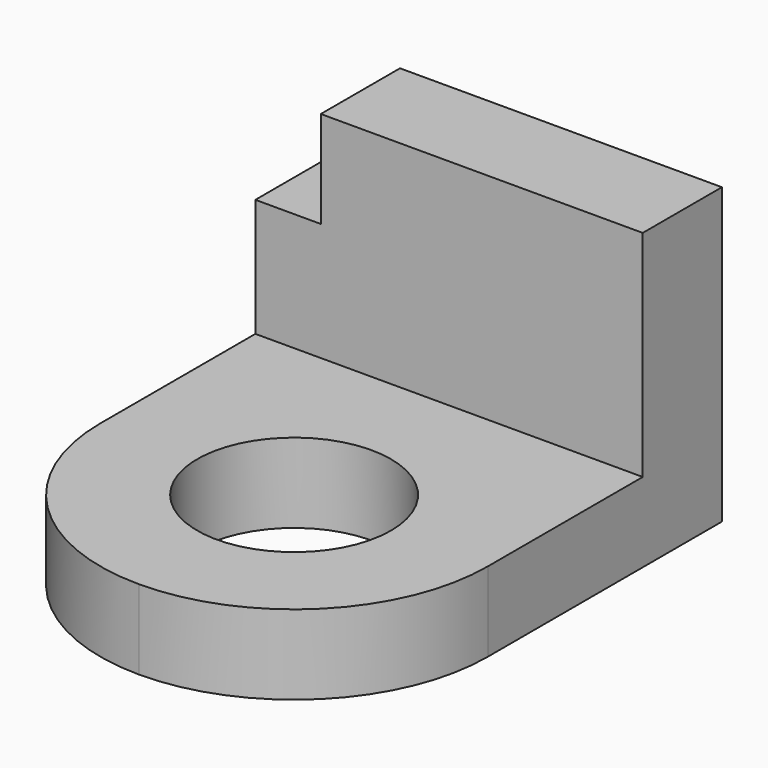
from build123d import *

# Parameters (mm, degrees)
F0_W     = 12.9794
F0_H     = 25.908
F1_DEPTH = 25.4
F2_W     = 42.2184414506
F2_H     = 12.9794
F3_DEPTH = 12.7
F4_W     = 50.8
F4_H     = 10.4306445336
F5_DEPTH = 50.8
F6_R     = 12.7
F7_DEPTH = 10.4316445336
F8_R     = 25.4
F9_R     = 25.39999


# Not quite as in the source:
# - a fillet or chamfer is up to 0.001 mm smaller than in the source, because OpenCascade refuses the exact size


with BuildPart() as f1:
    # F0 (on Right) → F1 (new body, symmetric)
    with BuildSketch(Plane.YZ):
        with Locations((35.6550812721, 2.5243262509)):
            Rectangle(F0_W, F0_H)
    extrude(amount=F1_DEPTH, both=True)

    # F2 (on face) → F3 (join)
    with BuildSketch(Plane.XY.offset(15.4783262509)):
        with Locations((4.2907792747, 35.6550812721)):
            Rectangle(F2_W, F2_H)
    extrude(amount=F3_DEPTH)

    # F4 (on face) → F5 (join)
    with BuildSketch(Plane.XZ.offset(-29.1653812721)):
        with Locations((0, -5.2143514823)):
            Rectangle(F4_W, F4_H)
    extrude(amount=F5_DEPTH)

    # F6 (on face) → F7 (cut, through all)
    with BuildSketch(Plane.XY.offset(0.0009707845)):
        with Locations((0, 3.7653812721)):
            Circle(F6_R)
    extrude(amount=-F7_DEPTH, mode=Mode.SUBTRACT)

    # F8
    f8_edges = [f1.edges().sort_by_distance(p)[0] for p in [
        (-25.4, -21.634619, -5.214351),
    ]]
    fillet(f8_edges, radius=F8_R)

    # F9 (radius 25.4 in the source; OpenCascade refuses exactly that, so slightly less here)
    f9_edges = [f1.edges().sort_by_distance(p)[0] for p in [
        (25.4, -21.634619, -5.214351),
    ]]
    fillet(f9_edges, radius=F9_R)


solid = f1.part
